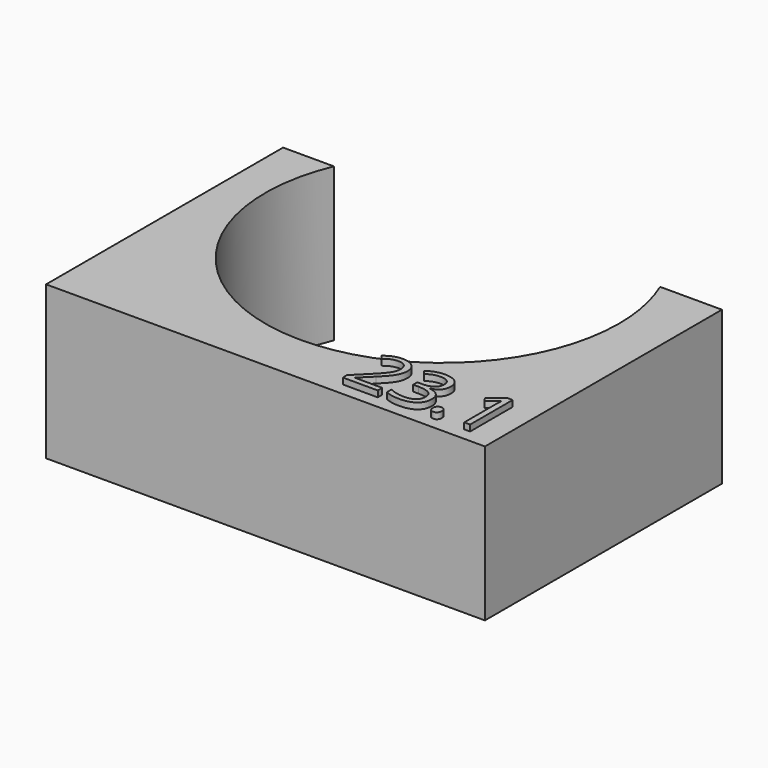
from build123d import *

# Parameters (mm, degrees)
F1_DEPTH     = 10
F4_TEXT_SIZE = 4.8614145877
F5_DEPTH     = 0.4


# Not quite as in the source:
# - Text() gives the source's letters only with a copy of the font that has no kerning and outlines rounded to 1/6400 em; it was checked with that copy


with BuildPart() as f1:
    # F0 (on Top) → F1 (new body)
    with BuildSketch(Plane.XY):
        with BuildLine():
            ThreePointArc((10.6470168996, 4.477000239), (11.3220039125, 2.2835777642), (11.55, 0))
            ThreePointArc((11.55, 0), (-2.2835777642, -11.3220039125), (-10.6470168996, 4.477000239))
            Line((-10.6470168996, 4.477000239), (-13.9682388768, 4.477000239))
            Line((-13.9682388768, 4.477000239), (-13.9682388768, -14.8636397033))
            Line((-13.9682388768, -14.8636397033), (14.6845622637, -14.8636397033))
            Line((14.6845622637, -14.8636397033), (14.6845622637, 4.477000239))
            Line((14.6845622637, 4.477000239), (10.6470168996, 4.477000239))
        make_face()
    extrude(amount=F1_DEPTH)


with BuildPart() as f2_1:
    # F2: copy of F1
    add(f1.part)


with BuildPart() as f1_1:
    add(f1.part)

    # F4 (on face) → F5 (join)
    with BuildSketch(Plane.XY.offset(10)):
        with Locations((4.5137116686, -14.0461027622)):
            Text('23.1', F4_TEXT_SIZE, font='Open Sans', text_align=(TextAlign.LEFT, TextAlign.BOTTOM))
    extrude(amount=F5_DEPTH)


solid = f1_1.part
